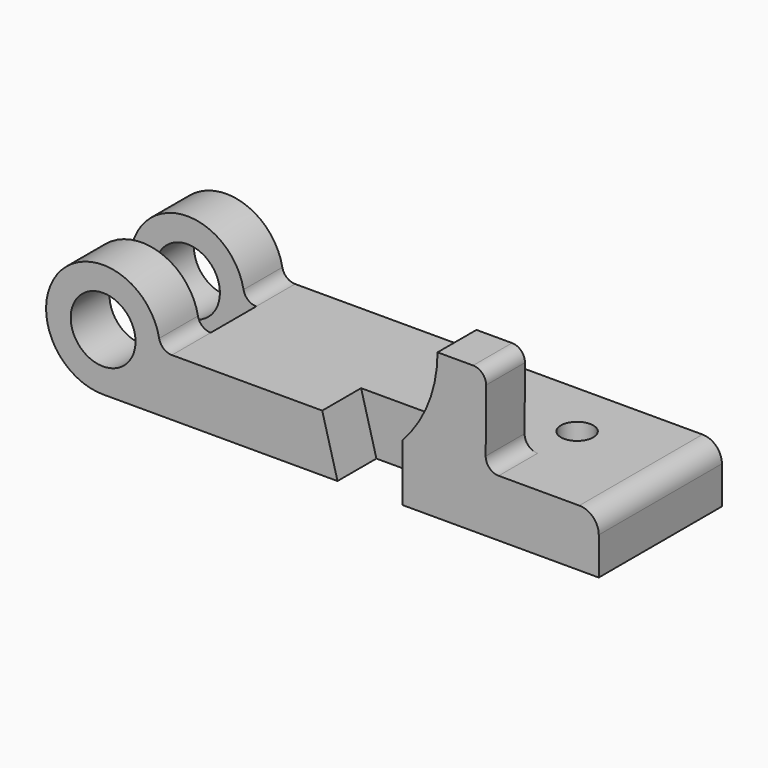
from build123d import *

# Parameters (mm, degrees)
F0_R      = 12.7
F1_DEPTH  = 30.1625
F4_R      = 5.08
F5_R      = 7.62
F6_R      = 5.08
F7_DEPTH  = 41.275
F9_DEPTH  = 19.05
F10_R     = 5.08
F11_W     = 22.352
F11_H     = 22.3266
F11_W_2   = 21.9653917967
F11_W_3   = 4.9921344993
F12_DEPTH = 57.151
F13_R     = 6.35
F14_DEPTH = 22.353


# Not quite as in the source:
# - a feature names something its author has since deleted; it is built from what else it names


with BuildPart() as f1:
    # F0 (on Front) → F1 (new body, symmetric)
    with BuildSketch(Plane.XZ):
        with BuildLine():
            Line((11.6077999467, 0), (5.6133999467, 22.352))
            Line((5.6133999467, 22.352), (-57.8866000533, 22.352))
            ThreePointArc((-57.8866000533, 22.352), (-64.4333492802, 6.5467492269), (-80.2386000533, 0))
            Line((-80.2386000533, 0), (11.6077999467, 0))
        make_face()
        Polygon((69.6339349389, 22.352), (37.0077999467, 22.352), (37.0077999467, 0), (69.4951486566, 0), align=None)
        Polygon((113.9697999467, 22.352), (69.6339349389, 22.352), (69.4951486566, 0), (113.9697999467, 0), align=None)
        with BuildLine():
            ThreePointArc((-80.2386000533, 0), (-64.4333492802, 6.5467492269), (-57.8866000533, 22.352))
            ThreePointArc((-57.8866000533, 22.352), (-96.0438508264, 38.1572507731), (-80.2386000533, 0))
        make_face()
        with Locations((-80.2386000533, 22.352)):
            Circle(F0_R, mode=Mode.SUBTRACT)
        Polygon((37.0077999467, 0), (37.0077999467, 22.352), (5.6133999467, 22.352), (11.6077999467, 0), align=None)
        with BuildLine():
            ThreePointArc((50.7999999467, 57.15), (47.2258153083, 38.4343576341), (37.0077999467, 22.352))
            Line((37.0077999467, 22.352), (69.6339349389, 22.352))
            Line((69.6339349389, 22.352), (69.8499999467, 57.15))
            Line((69.8499999467, 57.15), (50.7999999467, 57.15))
        make_face()
    extrude(amount=F1_DEPTH, both=True)

    # F4
    f4_edges = [f1.edges().sort_by_distance(p)[0] for p in [
        (69.85, 0, 57.15),
    ]]
    fillet(f4_edges, radius=F4_R)

    # F5
    f5_edges = [f1.edges().sort_by_distance(p)[0] for p in [
        (113.9698, 0, 22.352),
    ]]
    fillet(f5_edges, radius=F5_R)

    # F6
    f6_edges = [f1.edges().sort_by_distance(p)[0] for p in [
        (-57.8866, 0, 22.352),
    ]]
    fillet(f6_edges, radius=F6_R)

    # F3 (on face) → F7 (cut)
    with BuildSketch(Plane(origin=(0, 30.1625, 0), x_dir=(-1, 0, 0), z_dir=(0, 1, 0))):
        with BuildLine():
            Line((-69.8499999467, 57.15), (-69.6339349389, 22.352))
            Line((-69.6339349389, 22.352), (-37.0077999467, 22.352))
            ThreePointArc((-37.0077999467, 22.352), (-47.2258153083, 38.4343576341), (-50.7999999467, 57.15))
            Line((-50.7999999467, 57.15), (-69.8499999467, 57.15))
        make_face()
    extrude(amount=-F7_DEPTH, mode=Mode.SUBTRACT)

    # F2 (on face) → F9 (cut)
    with BuildSketch(Plane.XZ.offset(30.1625)):
        Polygon((37.0077999467, 22.352), (5.6133999467, 22.352), (11.6077999467, 0), (37.0077999467, 0), align=None)
    extrude(amount=-F9_DEPTH, mode=Mode.SUBTRACT)

    # F10
    f10_edges = [f1.edges().sort_by_distance(p)[0] for p in [
        (69.633935, -20.6375, 22.352),
    ]]
    fillet(f10_edges, radius=F10_R)

    # F11 (on Top) → F12 (cut, through all)
    with BuildSketch(Plane.XY):
        with Locations((-91.4146000533, 0)):
            Rectangle(F11_W, F11_H)
        with Locations((-69.2559041549, 0)):
            Rectangle(F11_W_2, F11_H)
        with Locations((-55.7771410069, 0)):
            Rectangle(F11_W_3, F11_H)
    extrude(amount=F12_DEPTH, mode=Mode.SUBTRACT)

    # F13 (on face) → F14 (cut, through all)
    with BuildSketch(Plane.XY.offset(22.352)):
        with Locations((75.1077999467, 7.8105)):
            Circle(F13_R)
    extrude(amount=-F14_DEPTH, mode=Mode.SUBTRACT)


solid = f1.part
